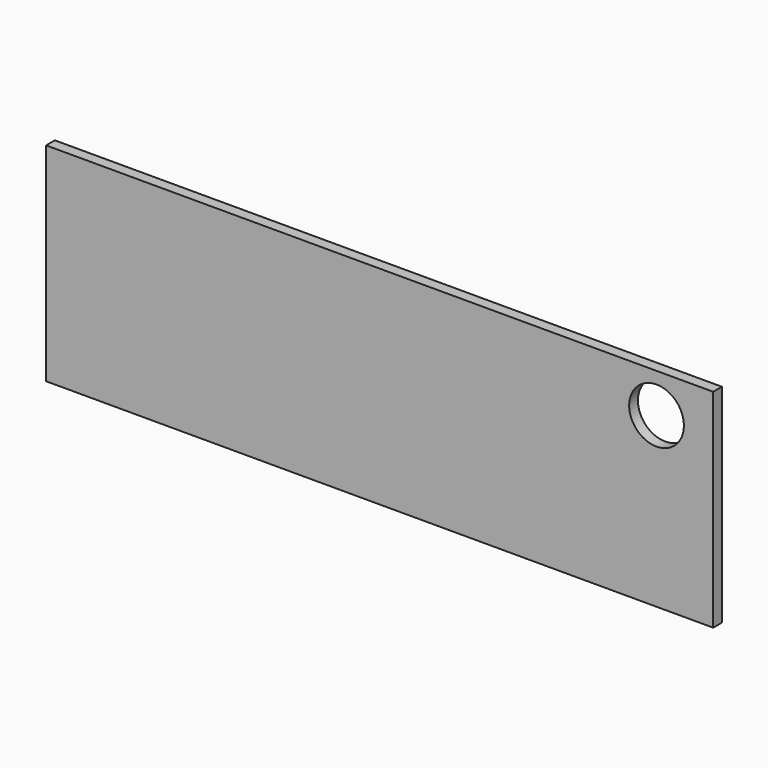
from build123d import *

# Parameters (mm, degrees)
F0_W           = 122.0296397805
F0_H           = 37.9903614521
F3_DEPTH       = 2
F5_D           = 10
F5_CBORE_D     = 10.0076
F5_CBORE_DEPTH = 5


# Not quite as in the source:
# - the program builds the solid bodies; features that only make, move or delete a surface that nothing else refers to are left out


with BuildPart() as f3:
    # F0 (on Front) → F3 (new body)
    with BuildSketch(Plane.XZ):
        Rectangle(F0_W, F0_H)
    extrude(amount=F3_DEPTH)

    # F5 (through all)
    with Locations(Plane(origin=(0, 0, 0), x_dir=(1, 0, 0), z_dir=(0, 1, 0))):
        with Locations((50.6538115442, -11.8000358343)):
            CounterBoreHole(F5_D / 2, F5_CBORE_D / 2, F5_CBORE_DEPTH)


solid = f3.part
